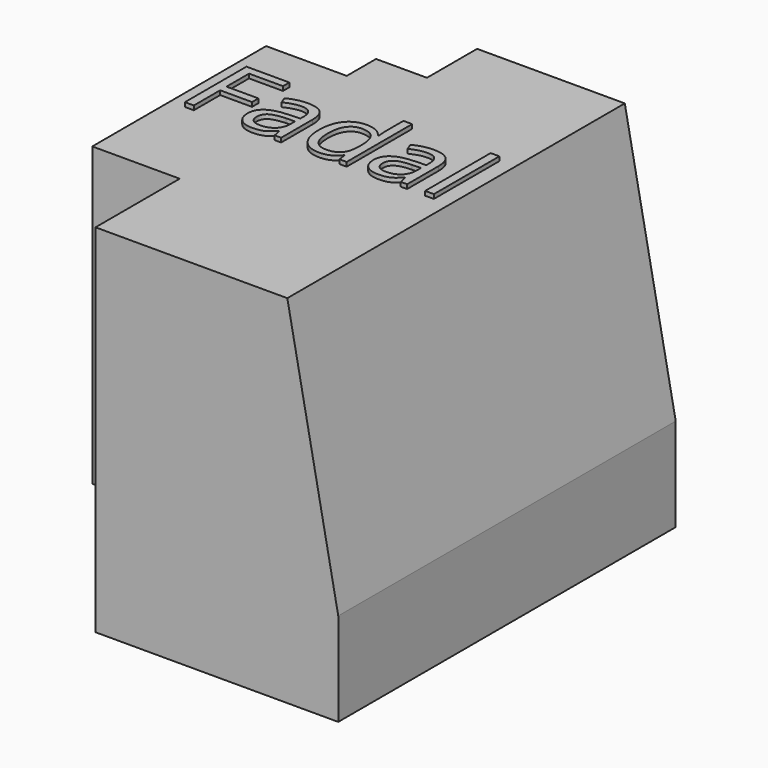
from build123d import *

# Parameters (mm, degrees)
F1_DEPTH     = 2100
F3_DEPTH     = 2485.001
F4_W         = 515
F4_H         = 350
F5_DEPTH     = 1865.001
F6_TEXT_SIZE = 634.8644721046
F7_DEPTH     = 25


# Not quite as in the source:
# - Text() gives the source's letters only with a copy of the font that has no kerning and outlines rounded to 1/6400 em; it was checked with that copy


with BuildPart() as f1:
    # F0 (on Top) → F1 (new body)
    with BuildSketch(Plane.XY):
        Polygon((-1430, 0), (0, 0), (0, 2485), (-1170, 2485), (-1170, 2115.7155036926), (-1470, 2115.7155036926), (-1470, 1900), (-1945, 1900), (-1945, 620), (-1430, 620), align=None)
    extrude(amount=F1_DEPTH)

    # F2 (on face) → F3 (cut, through all)
    with BuildSketch(Plane.XZ):
        Polygon((-300, 2100), (0, 550), (0, 2100), align=None)
    extrude(amount=-F3_DEPTH, mode=Mode.SUBTRACT)

    # F4 (on face) → F5 (cut, through all)
    with BuildSketch(Plane.XZ.offset(-620)):
        with Locations((-1687.5, 175)):
            Rectangle(F4_W, F4_H)
    extrude(amount=-F5_DEPTH, mode=Mode.SUBTRACT)

    # F6 (on face) → F7 (join)
    with BuildSketch(Plane.XY.offset(2100)):
        with Locations((-1920, 1192.8975800847)):
            Text('Fadal', F6_TEXT_SIZE, font='Open Sans', text_align=(TextAlign.LEFT, TextAlign.BOTTOM))
    extrude(amount=F7_DEPTH)


solid = f1.part
